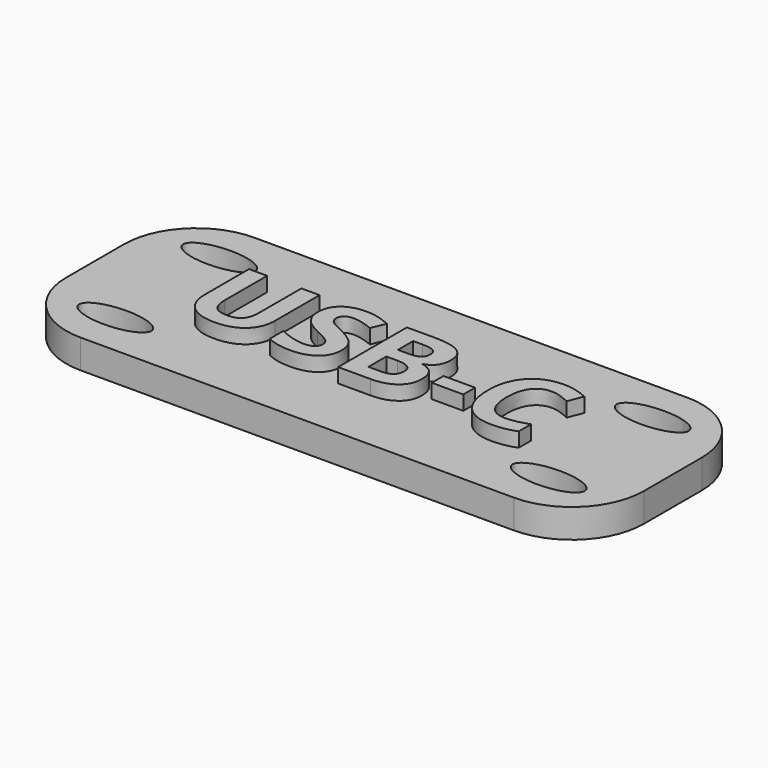
from build123d import *

# Parameters (mm, degrees)
F0_W         = 40
F0_H         = 15
F1_DEPTH     = 2
F2_TEXT_SIZE = 8.3333333333
F3_DEPTH     = 1
F4_R         = 5


# Not quite as in the source:
# - Text() gives the source's letters only with a copy of the font that has no kerning and outlines rounded to 1/6400 em; it was checked with that copy


with BuildPart() as f1:
    # F0 (on Top) → F1 (new body)
    with BuildSketch(Plane.XY):
        Rectangle(F0_W, F0_H)
        with BuildLine():
            add(Edge.make_bspline(
                [(-12.5, -4.5), (-12.5, -2.7679491924), (-16.25, -3.6339745962), (-20, -4.5), (-16.25, -5.3660254038), (-12.5, -6.2320508076), (-12.5, -4.5)],
                knots=[0, 0, 0, 2.0943951024, 2.0943951024, 4.1887902048, 4.1887902048, 6.2831853072, 6.2831853072, 6.2831853072], degree=2, weights=[1, 0.5, 1, 0.5, 1, 0.5, 1]))
        make_face(mode=Mode.SUBTRACT)
        with BuildLine():
            add(Edge.make_bspline(
                [(17.5, -4.5), (17.5, -2.7679491924), (13.75, -3.6339745962), (10, -4.5), (13.75, -5.3660254038), (17.5, -6.2320508076), (17.5, -4.5)],
                knots=[0, 0, 0, 2.0943951024, 2.0943951024, 4.1887902048, 4.1887902048, 6.2831853072, 6.2831853072, 6.2831853072], degree=2, weights=[1, 0.5, 1, 0.5, 1, 0.5, 1]))
        make_face(mode=Mode.SUBTRACT)
        with BuildLine():
            add(Edge.make_bspline(
                [(-12.5, 4.5), (-12.5, 6.2320508076), (-16.25, 5.3660254038), (-20, 4.5), (-16.25, 3.6339745962), (-12.5, 2.7679491924), (-12.5, 4.5)],
                knots=[0, 0, 0, 2.0943951024, 2.0943951024, 4.1887902048, 4.1887902048, 6.2831853072, 6.2831853072, 6.2831853072], degree=2, weights=[1, 0.5, 1, 0.5, 1, 0.5, 1]))
        make_face(mode=Mode.SUBTRACT)
        with BuildLine():
            add(Edge.make_bspline(
                [(17.5, 4.5), (17.5, 6.2320508076), (13.75, 5.3660254038), (10, 4.5), (13.75, 3.6339745962), (17.5, 2.7679491924), (17.5, 4.5)],
                knots=[0, 0, 0, 2.0943951024, 2.0943951024, 4.1887902048, 4.1887902048, 6.2831853072, 6.2831853072, 6.2831853072], degree=2, weights=[1, 0.5, 1, 0.5, 1, 0.5, 1]))
        make_face(mode=Mode.SUBTRACT)
    extrude(amount=F1_DEPTH)

    # F4
    f4_edges = [f1.edges().sort_by_distance(p)[0] for p in [
        (-20, -7.5, 1),
        (20, -7.5, 1),
        (20, 7.5, 1),
        (-20, 7.5, 1),
    ]]
    fillet(f4_edges, radius=F4_R)


with BuildPart() as f3:
    # F2 (on face) → F3 (new body)
    with BuildSketch(Plane.XY.offset(2)):
        with Locations((-12.4122792528, -3)):
            Text('USB-C', F2_TEXT_SIZE, font='Open Sans', font_style=FontStyle.BOLD, text_align=(TextAlign.LEFT, TextAlign.BOTTOM))
    extrude(amount=F3_DEPTH)


solid = Compound([f1.part, f3.part])
